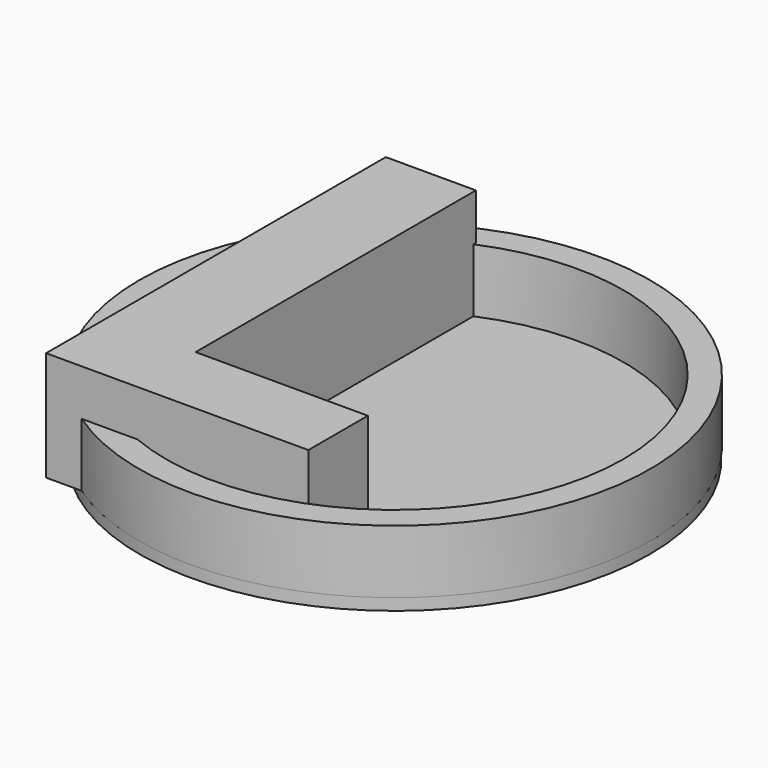
from build123d import *

# Parameters (mm, degrees)
F0_R         = 49.1675906864
F0_R_2       = 44.0180378732
F3_DEPTH     = 12.192
F1_TEXT_SIZE = 114.4279363669
F4_DEPTH     = 21.082
F6_R         = 49.0651918765
F7_DEPTH     = 2.286


# Not quite as in the source:
# - the program builds the solid bodies; features that only make, move or delete a surface that nothing else refers to are left out
# - Text() gives the source's letters only with a copy of the font that has no kerning and outlines rounded to 1/6400 em; it was checked with that copy


with BuildPart() as f3:
    # F0 (on Top) → F3 (new body)
    with BuildSketch(Plane.XY):
        Circle(F0_R)
        Circle(F0_R_2, mode=Mode.SUBTRACT)
    extrude(amount=F3_DEPTH)

    # F1 (on face) → F4 (join)
    with BuildSketch(Plane.XY):
        with Locations((-44.8611695319, -40.604647249)):
            Text('L', F1_TEXT_SIZE, font='Open Sans', font_style=FontStyle.BOLD, text_align=(TextAlign.LEFT, TextAlign.BOTTOM))
    extrude(amount=F4_DEPTH)

    # F6 (on Top) → F7 (join)
    with BuildSketch(Plane.XY):
        Circle(F6_R)
    extrude(amount=-F7_DEPTH)


solid = f3.part
